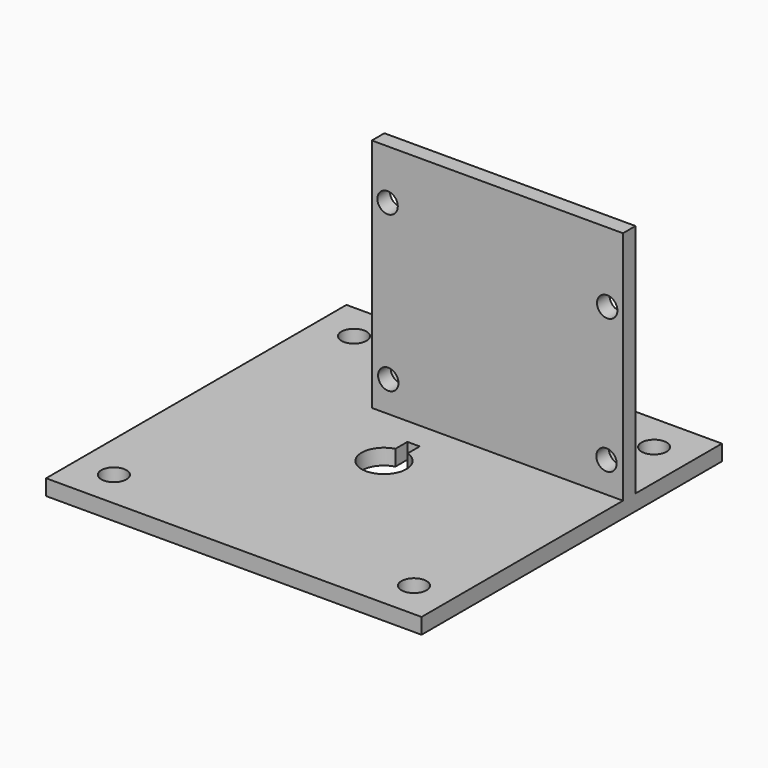
from build123d import *

# Parameters (mm, degrees)
F0_R     = 2
F1_DEPTH = 2.5
F2_DEPTH = 40
F3_R     = 1.625
F4_DEPTH = 25


# Not quite as in the source:
# - a feature names something its author has since deleted; it is built from what else it names


with BuildPart() as f1:
    # F0 (on Top) → F1 (new body)
    with BuildSketch(Plane.XY):
        Polygon((29.9, 29.9), (-29.9, 29.9), (-29.9, -29.9), (29.9, -29.9), (29.9, 10.2), (1.0269208253, 10.2), (0.8924006252, 10.2), (-0.932000461, 10.2), (-10.1, 10.2), (-10.1, 12.7), (29.9, 12.7), align=None)
        with Locations((-23.9, -23.9)):
            Circle(F0_R, mode=Mode.SUBTRACT)
        with Locations((23.9, -23.9)):
            Circle(F0_R, mode=Mode.SUBTRACT)
        with BuildLine():
            ThreePointArc((1.0269208253, 3.4086703593), (2.8573972543, 2.1234125673), (3.56, 0))
            ThreePointArc((3.56, 0), (-2.1628312878, -2.8276776373), (-0.932000461, 3.4358368909))
            Line((-0.932000461, 3.4358368909), (-0.932000461, 5.8278255165))
            Line((-0.932000461, 5.8278255165), (1.0269208253, 5.8278255165))
            Line((1.0269208253, 5.8278255165), (1.0269208253, 3.4086703593))
        make_face(mode=Mode.SUBTRACT)
        with Locations((-23.9, 23.9)):
            Circle(F0_R, mode=Mode.SUBTRACT)
        with Locations((23.9, 23.9)):
            Circle(F0_R, mode=Mode.SUBTRACT)
    extrude(amount=F1_DEPTH)

    # F0 (on Top) → F2 (join)
    with BuildSketch(Plane.XY):
        Polygon((29.9, 10.2), (29.9, 12.7), (-10.1, 12.7), (-10.1, 10.2), (-0.932000461, 10.2), (0.8924006252, 10.2), (1.0269208253, 10.2), align=None)
    extrude(amount=F2_DEPTH)

    # F3 (on face) → F4 (cut)
    with BuildSketch(Plane.XZ.offset(-10.2)):
        with Locations((-7.5884815305, 32.100006938)):
            Circle(F3_R)
        with Locations((-7.475, 7.375)):
            Circle(F3_R)
        with Locations((27.3884814233, 28.875)):
            Circle(F3_R)
        with Locations((27.275, 7.375)):
            Circle(F3_R)
    extrude(amount=-F4_DEPTH, mode=Mode.SUBTRACT)


solid = f1.part
